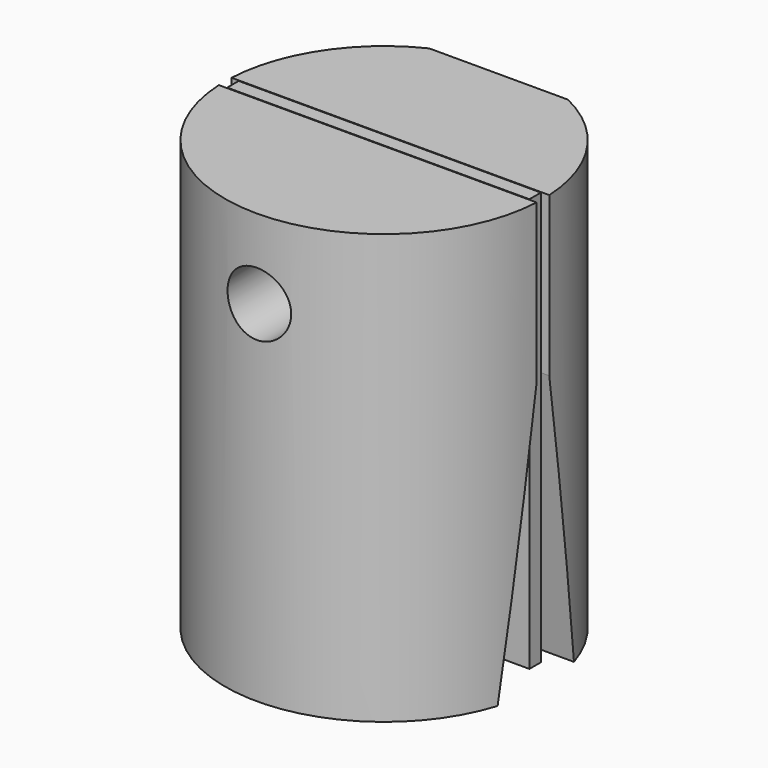
from build123d import *

# Parameters (mm, degrees)
F0_R      = 10
F1_DEPTH  = 25
F3_DEPTH  = 12.5
F4_DEPTH  = 10
F6_DEPTH  = 12.5
F7_R      = 2
F8_DEPTH  = 12.5
F9_W      = 19
F9_H      = 0.9
F10_DEPTH = 26
F11_W     = 62.5739917159
F11_H     = 29.2480699718
F12_DEPTH = 30


with BuildPart() as f1:
    # F0 (on Top) → F1 (new body)
    with BuildSketch(Plane.XY):
        Circle(F0_R)
    extrude(amount=F1_DEPTH)

    # F2 (on Right) → F3 (cut, symmetric)
    with BuildSketch(Plane.YZ):
        Polygon((-3, 8), (3, 8), (0.5, 25), (-0.5, 25), align=None)
    extrude(amount=F3_DEPTH, both=True, mode=Mode.SUBTRACT)

    # F4 (add): faces of the model
    f4_faces = [f1.faces().sort_by_distance(p)[0] for p in [
        (0, 4.5155770092, 25),
        (0, -4.5155770092, 25),
    ]]
    extrude(f4_faces, amount=F4_DEPTH)

    # F5 (on Right) → F6 (cut, symmetric)
    with BuildSketch(Plane.YZ):
        Polygon((29.1443374008, 8), (-21.5125791728, 8), (-21.9593886286, -11.827128388), (29.8704002053, -10.9335111063), align=None)
    extrude(amount=F6_DEPTH, both=True, mode=Mode.SUBTRACT)

    # F7 (on Front) → F8 (cut, symmetric)
    with BuildSketch(Plane.XZ):
        with Locations((0, 30)):
            Circle(F7_R)
    extrude(amount=F8_DEPTH, both=True, mode=Mode.SUBTRACT)

    # F11 (on face) → F12 (cut)
    with BuildSketch(Plane(origin=(0, 0, 8), x_dir=(1, 0, 0), z_dir=(0, 0, -1))):
        with Locations((3.5222135484, 0.1944573596)):
            Rectangle(F11_W, F11_H)
        with BuildLine():
            Line((19.6776342417, -9), (-17.8668759763, -9))
            Line((-17.8668759763, -9), (-17.8668759763, 9))
            Line((-17.8668759763, 9), (-4.3588989435, 9))
            ThreePointArc((-4.3588989435, 9), (0, 10), (4.3588989435, 9))
            Line((4.3588989435, 9), (19.6776342417, 9))
            Line((19.6776342417, 9), (19.6776342417, -9))
        make_face(mode=Mode.SUBTRACT)
    extrude(amount=-F12_DEPTH, mode=Mode.SUBTRACT)


with BuildPart() as f10:
    # F9 (on face) → F10 (new body)
    with BuildSketch(Plane.XY.offset(35)):
        Rectangle(F9_W, F9_H)
    extrude(amount=-F10_DEPTH)


solid = Compound([f1.part, f10.part])
